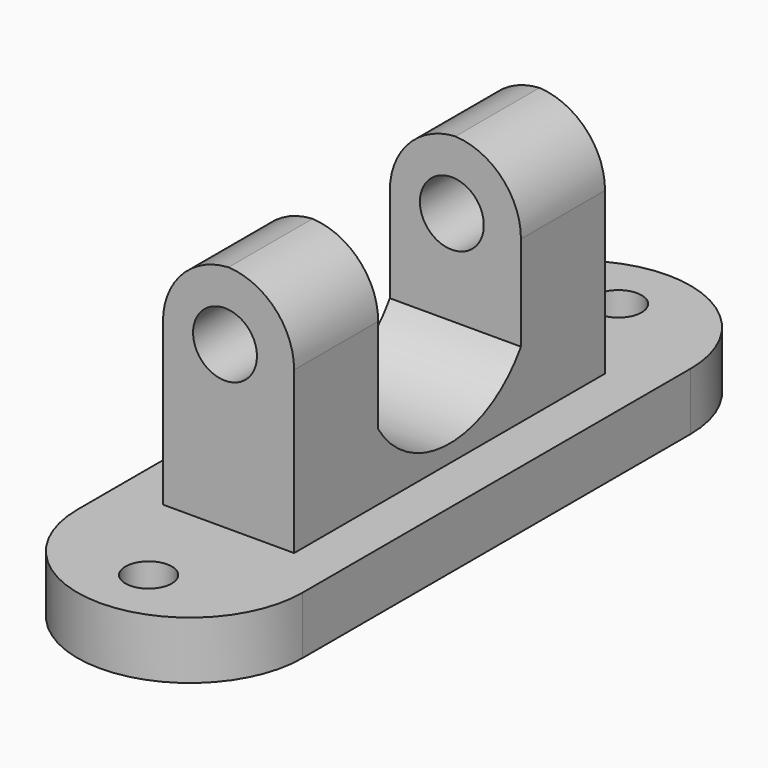
from build123d import *

# Parameters (mm, degrees)
F0_R          = 5.1422573348
F0_W          = 49.6318712831
F0_H          = 106.9652438164
F0_R_2        = 5.1025471004
F1_DEPTH      = 12.7
F2_W          = 28.9213098586
F2_H          = 85.7132077217
F3_DEPTH      = 50.8
F4_T1_DEPTH   = 161.9132077217
F5_R          = 7.0462908342
F6_DEPTH      = 101.6
F7_W          = 39.3632203341
F7_H          = 41.8217248726
F8_DEPTH      = 50.8
F8_DEPTH_BACK = 25.4


# Not quite as in the source:
# - a fillet or chamfer that OpenCascade refuses, or shapes differently, is made with other operations: its cross-section is extruded or revolved along the edge and cut away or added


with BuildPart() as f1:
    # F0 (on Top) → F1 (new body)
    with BuildSketch(Plane.XY):
        with BuildLine():
            ThreePointArc((24.8159356415, 53.4826219082), (0, 78.2985575497), (-24.8159356415, 53.4826219082))
            Line((-24.8159356415, 53.4826219082), (24.8159356415, 53.4826219082))
        make_face()
        with Locations((0, 64.6070018411)):
            Circle(F0_R, mode=Mode.SUBTRACT)
        Rectangle(F0_W, F0_H)
        with BuildLine():
            Line((24.8159356415, -53.4826219082), (-24.8159356415, -53.4826219082))
            ThreePointArc((-24.8159356415, -53.4826219082), (0, -78.2985575497), (24.8159356415, -53.4826219082))
        make_face()
        with Locations((0, -64.8922473192)):
            Circle(F0_R_2, mode=Mode.SUBTRACT)
    extrude(amount=F1_DEPTH)

    # F2 (on face) → F3 (join)
    with BuildSketch(Plane.XY.offset(12.7)):
        Rectangle(F2_W, F2_H)
    extrude(amount=F3_DEPTH)

    # F4: fillet of radius 15.24 on 2 edges, made by hand

    # F4_s2 → F4_t1 (cut)
    with BuildSketch(Plane.XZ.offset(-80.9566038609)):
        with BuildLine():
            ThreePointArc((14.4606549293, 48.26), (9.9969622746, 59.0363073453), (-0.7793450707, 63.5))
            Line((-0.7793450707, 63.5), (14.4606549293, 63.5))
            Line((14.4606549293, 63.5), (14.4606549293, 48.26))
        make_face()
        with BuildLine():
            ThreePointArc((-14.4606549293, 48.26), (-9.9969622746, 59.0363073453), (0.7793450707, 63.5))
            Line((0.7793450707, 63.5), (-14.4606549293, 63.5))
            Line((-14.4606549293, 63.5), (-14.4606549293, 48.26))
        make_face()
    extrude(amount=F4_T1_DEPTH, mode=Mode.SUBTRACT)

    # F5 (on face) → F6 (cut)
    with BuildSketch(Plane(origin=(0, 42.8566038609, 0), x_dir=(-1, 0, 0), z_dir=(0, 1, 0))):
        with Locations((0.7793450707, 48.26)):
            Circle(F5_R)
    extrude(amount=-F6_DEPTH, mode=Mode.SUBTRACT)

    # F7 (on face) → F8 (cut, two sides)
    with BuildSketch(Plane(origin=(-14.4606549293, 0, 0), x_dir=(0, -1, 0), z_dir=(-1, 0, 0))) as f8_sk:
        with Locations((0, 48.26)):
            Rectangle(F7_W, F7_H)
        with BuildLine():
            Line((19.681610167, 27.3491375637), (-19.681610167, 27.3491375637))
            ThreePointArc((-19.681610167, 27.3491375637), (0, 16.517771495), (19.681610167, 27.3491375637))
        make_face()
    extrude(amount=-F8_DEPTH, mode=Mode.SUBTRACT)
    extrude(f8_sk.sketch, amount=F8_DEPTH_BACK, mode=Mode.SUBTRACT)


solid = f1.part
